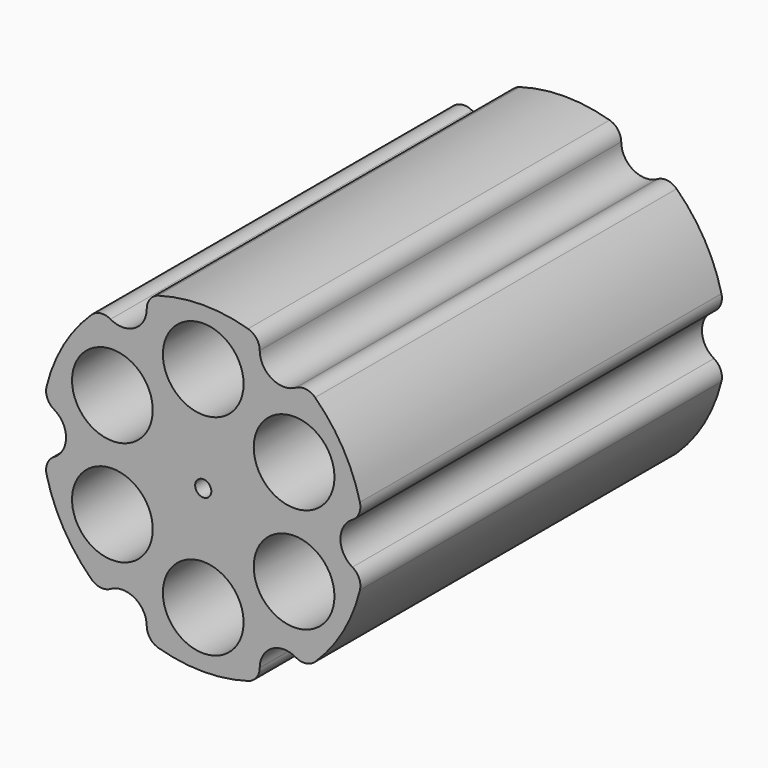
from build123d import *

# Parameters (mm, degrees)
F0_R             = 31.75
F1_DEPTH         = 88.9
F2_R             = 7.9375
F3_DEPTH         = 20.6375
F3_COPIES_COUNT  = 6
F4_R             = 6.35
F5_DEPTH         = 55.626
F5_TAPER         = 0.375
F5_COPIES_COUNT  = 6
F6_R             = 1.5875
F7_DEPTH         = 88.901
F8_R             = 9.525
F9_DEPTH         = 12.6375
F9_COPIES_COUNT  = 6
F10_R            = 4.7625
F11_DEPTH        = 88.901
F11_COPIES_COUNT = 6
F12_R            = 3.175


# Not quite as in the source:
# - a pattern or mirror of a feature is missing from the dataset's text; its kind, count and spacing are read off the source's solid


with BuildPart() as f1:
    # F0 (on Front) → F1 (new body)
    with BuildSketch(Plane.XZ):
        Circle(F0_R)
    extrude(amount=F1_DEPTH)

    # F2 (on face) → F3 (cut)
    with BuildSketch(Plane.XZ.offset(88.9)):
        with Locations((0, 20.6375)):
            Circle(F2_R)
    f3 = extrude(amount=-F3_DEPTH, mode=Mode.SUBTRACT)

    # F3_copies: F3 ×6 about axis
    f3_copies_axis = Axis((0, 0, 0), (0, 1, 0))
    for i in range(1, F3_COPIES_COUNT):
        add(f3.rotate(f3_copies_axis, i * 360 / F3_COPIES_COUNT), mode=Mode.SUBTRACT)

    # F4 (on face) → F5 (cut)
    with BuildSketch(Plane.XZ.offset(68.2625)):
        with Locations((0, 20.6375)):
            Circle(F4_R)
    f5 = extrude(amount=-F5_DEPTH, taper=F5_TAPER, mode=Mode.SUBTRACT)

    # F5_copies: F5 ×6 about axis
    f5_copies_axis = Axis((0, 0, 0), (0, 1, 0))
    for i in range(1, F5_COPIES_COUNT):
        add(f5.rotate(f5_copies_axis, i * 360 / F5_COPIES_COUNT), mode=Mode.SUBTRACT)

    # F6 (on face) → F7 (cut, through all)
    with BuildSketch(Plane.XZ.offset(88.9)):
        Circle(F6_R)
    extrude(amount=-F7_DEPTH, mode=Mode.SUBTRACT)

    # F8 (on face) → F9 (cut, through all)
    with BuildSketch(Plane.XZ.offset(12.6365)):
        with Locations((0, 20.6375)):
            Circle(F8_R)
    f9 = extrude(amount=-F9_DEPTH, mode=Mode.SUBTRACT)

    # F9_copies: F9 ×6 about axis
    f9_copies_axis = Axis((0, 0, 0), (0, 1, 0))
    for i in range(1, F9_COPIES_COUNT):
        add(f9.rotate(f9_copies_axis, i * 360 / F9_COPIES_COUNT), mode=Mode.SUBTRACT)

    # F10 (on face) → F11 (cut, through all)
    with BuildSketch(Plane.XZ.offset(88.9)):
        with Locations((-15.875, 27.4963065702)):
            Circle(F10_R)
    f11 = extrude(amount=-F11_DEPTH, mode=Mode.SUBTRACT)

    # F11_copies: F11 ×6 about axis
    f11_copies_axis = Axis((0, 0, 0), (0, 1, 0))
    for i in range(1, F11_COPIES_COUNT):
        add(f11.rotate(f11_copies_axis, i * 360 / F11_COPIES_COUNT), mode=Mode.SUBTRACT)

    # F12
    f12_edges = [f1.edges().sort_by_distance(p)[0] for p in [
        (-19.809236, -44.45, 24.81243),
        (-11.583577, -44.45, 29.561516),
        (-31.392813, -44.45, 4.749087),
        (11.583577, -44.45, 29.561516),
        (19.809236, -44.45, 24.81243),
        (31.392812, -44.45, 4.749087),
        (31.392813, -44.45, -4.749087),
        (19.809236, -44.45, -24.81243),
        (11.583577, -44.45, -29.561516),
        (-11.583577, -44.45, -29.561516),
        (-19.809236, -44.45, -24.81243),
        (-31.392813, -44.45, -4.749087),
    ]]
    fillet(f12_edges, radius=F12_R)


solid = f1.part
